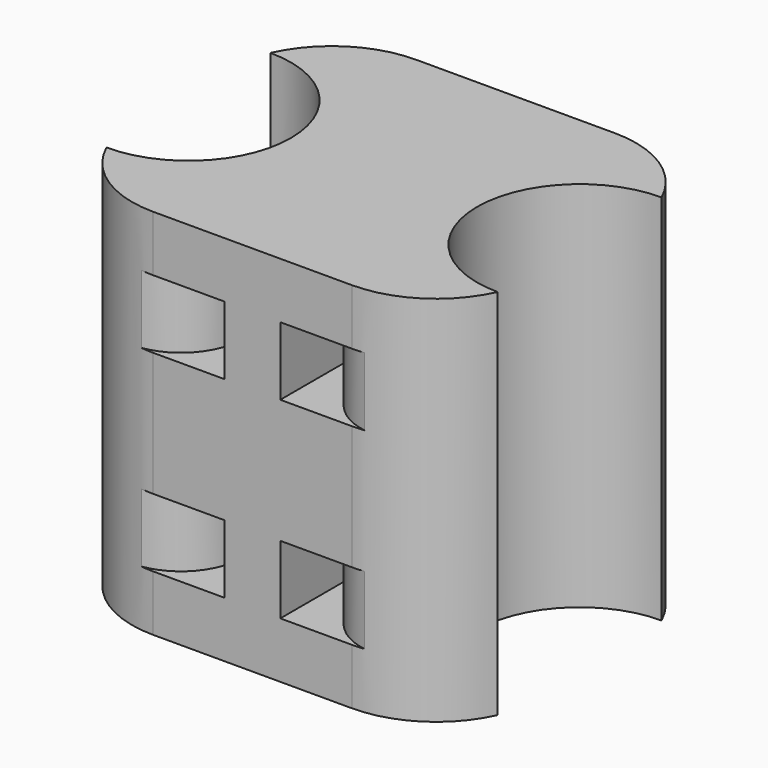
from build123d import *

# Parameters (mm, degrees)
F1_DEPTH     = 30
F2_W         = 2.5
F2_H         = 5.5
F3_DEPTH     = 27
F4_T1_DEPTH  = 68.7298334621
F5_T1_DEPTH  = 5.5
F5_T3_DEPTH  = 5.5
F5_T8_DEPTH  = 30.5
F5_T13_DEPTH = 30.5
F5_T18_DEPTH = 30.5
F5_T23_DEPTH = 30.5
F5_T28_DEPTH = 30.5
F5_T33_DEPTH = 30.5
F5_T38_DEPTH = 30.5
F5_T43_DEPTH = 30.5


# Not quite as in the source:
# - a fillet or chamfer that OpenCascade refuses, or shapes differently, is made with other operations: its cross-section is extruded or revolved along the edge and cut away or added


with BuildPart() as f1:
    # F0 (on Top) → F1 (new body)
    with BuildSketch(Plane.XY):
        with BuildLine():
            Line((15.75, 13.25), (-15.75, 13.25))
            Line((-15.75, 13.25), (-15.75, 8.25))
            ThreePointArc((-15.75, 8.25), (-9.9163690552, 5.8336309448), (-7.5, 0))
            ThreePointArc((-7.5, 0), (-9.9163690552, -5.8336309448), (-15.75, -8.25))
            Line((-15.75, -8.25), (-15.75, -13.25))
            Line((-15.75, -13.25), (15.75, -13.25))
            Line((15.75, -13.25), (15.75, -8.25))
            ThreePointArc((15.75, -8.25), (7.5, 0), (15.75, 8.25))
            Line((15.75, 8.25), (15.75, 13.25))
        make_face()
    extrude(amount=F1_DEPTH)

    # F2 (on face) → F3 (cut)
    with BuildSketch(Plane.XZ.offset(13.25)):
        with Locations((-3.5, 22.75)):
            Rectangle(F2_W, F2_H)
        with Locations((-3.5, 7.25)):
            Rectangle(F2_W, F2_H)
        with Locations((3.5, 22.75)):
            Rectangle(F2_W, F2_H)
        with Locations((3.5, 7.25)):
            Rectangle(F2_W, F2_H)
    extrude(amount=-F3_DEPTH, mode=Mode.SUBTRACT)

    # F4: fillet of radius 8.5 on 4 edges, made by hand

    # F4_s2 → F4_t1 (cut)
    with BuildSketch(Plane.XY.offset(-19.364916731)):
        with BuildLine():
            ThreePointArc((-8.0040333076, 13.25), (-12.6138055362, 11.8914284285), (-15.75, 8.25))
            Line((-15.75, 8.25), (-15.75, 13.25))
            Line((-15.75, 13.25), (-8.0040333076, 13.25))
        make_face()
        with BuildLine():
            ThreePointArc((-8.0040333076, -13.25), (-12.6138055362, -11.8914284285), (-15.75, -8.25))
            Line((-15.75, -8.25), (-15.75, -13.25))
            Line((-15.75, -13.25), (-8.0040333076, -13.25))
        make_face()
        with BuildLine():
            ThreePointArc((15.75, -8.25), (12.6138055362, -11.8914284285), (8.0040333076, -13.25))
            Line((8.0040333076, -13.25), (15.75, -13.25))
            Line((15.75, -13.25), (15.75, -8.25))
        make_face()
        with BuildLine():
            ThreePointArc((15.75, 8.25), (12.6138055362, 11.8914284285), (8.0040333076, 13.25))
            Line((8.0040333076, 13.25), (15.75, 13.25))
            Line((15.75, 13.25), (15.75, 8.25))
        make_face()
    extrude(amount=F4_T1_DEPTH, mode=Mode.SUBTRACT)

    # F5: fillet of radius 5 on 8 edges, made by hand

    # F5_s2 → F5_t1 (cut)
    with BuildSketch(Plane.XY.offset(20)):
        with BuildLine():
            ThreePointArc((-9.75, -13.25), (-6.2144660941, -11.7855339059), (-4.75, -8.25))
            Line((-4.75, -8.25), (-4.75, -13.25))
            Line((-4.75, -13.25), (-9.75, -13.25))
        make_face()
        with BuildLine():
            ThreePointArc((9.75, -13.25), (6.2144660941, -11.7855339059), (4.75, -8.25))
            Line((4.75, -8.25), (4.75, -13.25))
            Line((4.75, -13.25), (9.75, -13.25))
        make_face()
        with BuildLine():
            ThreePointArc((9.75, 13.25), (6.2144660941, 11.7855339059), (4.75, 8.25))
            Line((4.75, 8.25), (4.75, 13.25))
            Line((4.75, 13.25), (9.75, 13.25))
        make_face()
        with BuildLine():
            ThreePointArc((-9.75, 13.25), (-6.2144660941, 11.7855339059), (-4.75, 8.25))
            Line((-4.75, 8.25), (-4.75, 13.25))
            Line((-4.75, 13.25), (-9.75, 13.25))
        make_face()
    extrude(amount=F5_T1_DEPTH, mode=Mode.SUBTRACT)

    # F5_s4 → F5_t3 (cut)
    with BuildSketch(Plane.XY.offset(4.5)):
        with BuildLine():
            ThreePointArc((-9.75, -13.25), (-6.2144660941, -11.7855339059), (-4.75, -8.25))
            Line((-4.75, -8.25), (-4.75, -13.25))
            Line((-4.75, -13.25), (-9.75, -13.25))
        make_face()
        with BuildLine():
            ThreePointArc((9.75, -13.25), (6.2144660941, -11.7855339059), (4.75, -8.25))
            Line((4.75, -8.25), (4.75, -13.25))
            Line((4.75, -13.25), (9.75, -13.25))
        make_face()
        with BuildLine():
            ThreePointArc((9.75, 13.25), (6.2144660941, 11.7855339059), (4.75, 8.25))
            Line((4.75, 8.25), (4.75, 13.25))
            Line((4.75, 13.25), (9.75, 13.25))
        make_face()
        with BuildLine():
            ThreePointArc((-9.75, 13.25), (-6.2144660941, 11.7855339059), (-4.75, 8.25))
            Line((-4.75, 8.25), (-4.75, 13.25))
            Line((-4.75, 13.25), (-9.75, 13.25))
        make_face()
    extrude(amount=F5_T3_DEPTH, mode=Mode.SUBTRACT)


with BuildPart() as f5_tool6:
    # F5_s7 → F5_t8 (new body)
    with BuildSketch(Plane.XY.offset(38)):
        with BuildLine():
            ThreePointArc((-9.75, -13.25), (-6.2144660941, -11.7855339059), (-4.75, -8.25))
            Line((-4.75, -8.25), (-4.75, -13.25))
            Line((-4.75, -13.25), (-9.75, -13.25))
        make_face()
    extrude(amount=-F5_T8_DEPTH)

    split(bisect_by=Plane.XY.offset(10), keep=Keep.BOTTOM)


with BuildPart() as f1_1:
    add(f1.part)

    # F5_t5: cut F5_tool6
    add(f5_tool6.part, mode=Mode.SUBTRACT)


with BuildPart() as f5_tool11:
    # F5_s12 → F5_t13 (new body)
    with BuildSketch(Plane.XY.offset(22.5)):
        with BuildLine():
            ThreePointArc((-9.75, -13.25), (-6.2144660941, -11.7855339059), (-4.75, -8.25))
            Line((-4.75, -8.25), (-4.75, -13.25))
            Line((-4.75, -13.25), (-9.75, -13.25))
        make_face()
    extrude(amount=-F5_T13_DEPTH)

    split(bisect_by=Plane.XY.offset(20), keep=Keep.TOP)


with BuildPart() as f1_2:
    add(f1_1.part)

    # F5_t10: cut F5_tool11
    add(f5_tool11.part, mode=Mode.SUBTRACT)


with BuildPart() as f5_tool16:
    # F5_s17 → F5_t18 (new body)
    with BuildSketch(Plane.XY.offset(7.5)):
        with BuildLine():
            ThreePointArc((9.75, -13.25), (6.2144660941, -11.7855339059), (4.75, -8.25))
            Line((4.75, -8.25), (4.75, -13.25))
            Line((4.75, -13.25), (9.75, -13.25))
        make_face()
    extrude(amount=F5_T18_DEPTH)

    split(bisect_by=Plane.XY.offset(10), keep=Keep.BOTTOM)


with BuildPart() as f1_3:
    add(f1_2.part)

    # F5_t15: cut F5_tool16
    add(f5_tool16.part, mode=Mode.SUBTRACT)


with BuildPart() as f5_tool21:
    # F5_s22 → F5_t23 (new body)
    with BuildSketch(Plane.XY.offset(-8)):
        with BuildLine():
            ThreePointArc((9.75, -13.25), (6.2144660941, -11.7855339059), (4.75, -8.25))
            Line((4.75, -8.25), (4.75, -13.25))
            Line((4.75, -13.25), (9.75, -13.25))
        make_face()
    extrude(amount=F5_T23_DEPTH)

    split(bisect_by=Plane.XY.offset(20), keep=Keep.TOP)


with BuildPart() as f1_4:
    add(f1_3.part)

    # F5_t20: cut F5_tool21
    add(f5_tool21.part, mode=Mode.SUBTRACT)


with BuildPart() as f5_tool26:
    # F5_s27 → F5_t28 (new body)
    with BuildSketch(Plane.XY.offset(7.5)):
        with BuildLine():
            ThreePointArc((9.75, 13.25), (6.2144660941, 11.7855339059), (4.75, 8.25))
            Line((4.75, 8.25), (4.75, 13.25))
            Line((4.75, 13.25), (9.75, 13.25))
        make_face()
    extrude(amount=F5_T28_DEPTH)

    split(bisect_by=Plane.XY.offset(10), keep=Keep.BOTTOM)


with BuildPart() as f1_5:
    add(f1_4.part)

    # F5_t25: cut F5_tool26
    add(f5_tool26.part, mode=Mode.SUBTRACT)


with BuildPart() as f5_tool31:
    # F5_s32 → F5_t33 (new body)
    with BuildSketch(Plane.XY.offset(-8)):
        with BuildLine():
            ThreePointArc((9.75, 13.25), (6.2144660941, 11.7855339059), (4.75, 8.25))
            Line((4.75, 8.25), (4.75, 13.25))
            Line((4.75, 13.25), (9.75, 13.25))
        make_face()
    extrude(amount=F5_T33_DEPTH)

    split(bisect_by=Plane.XY.offset(20), keep=Keep.TOP)


with BuildPart() as f1_6:
    add(f1_5.part)

    # F5_t30: cut F5_tool31
    add(f5_tool31.part, mode=Mode.SUBTRACT)


with BuildPart() as f5_tool36:
    # F5_s37 → F5_t38 (new body)
    with BuildSketch(Plane.XY.offset(38)):
        with BuildLine():
            ThreePointArc((-9.75, 13.25), (-6.2144660941, 11.7855339059), (-4.75, 8.25))
            Line((-4.75, 8.25), (-4.75, 13.25))
            Line((-4.75, 13.25), (-9.75, 13.25))
        make_face()
    extrude(amount=-F5_T38_DEPTH)

    split(bisect_by=Plane.XY.offset(10), keep=Keep.BOTTOM)


with BuildPart() as f1_7:
    add(f1_6.part)

    # F5_t35: cut F5_tool36
    add(f5_tool36.part, mode=Mode.SUBTRACT)


with BuildPart() as f5_tool41:
    # F5_s42 → F5_t43 (new body)
    with BuildSketch(Plane.XY.offset(22.5)):
        with BuildLine():
            ThreePointArc((-9.75, 13.25), (-6.2144660941, 11.7855339059), (-4.75, 8.25))
            Line((-4.75, 8.25), (-4.75, 13.25))
            Line((-4.75, 13.25), (-9.75, 13.25))
        make_face()
    extrude(amount=-F5_T43_DEPTH)

    split(bisect_by=Plane.XY.offset(20), keep=Keep.TOP)


with BuildPart() as f1_8:
    add(f1_7.part)

    # F5_t40: cut F5_tool41
    add(f5_tool41.part, mode=Mode.SUBTRACT)


solid = f1_8.part
